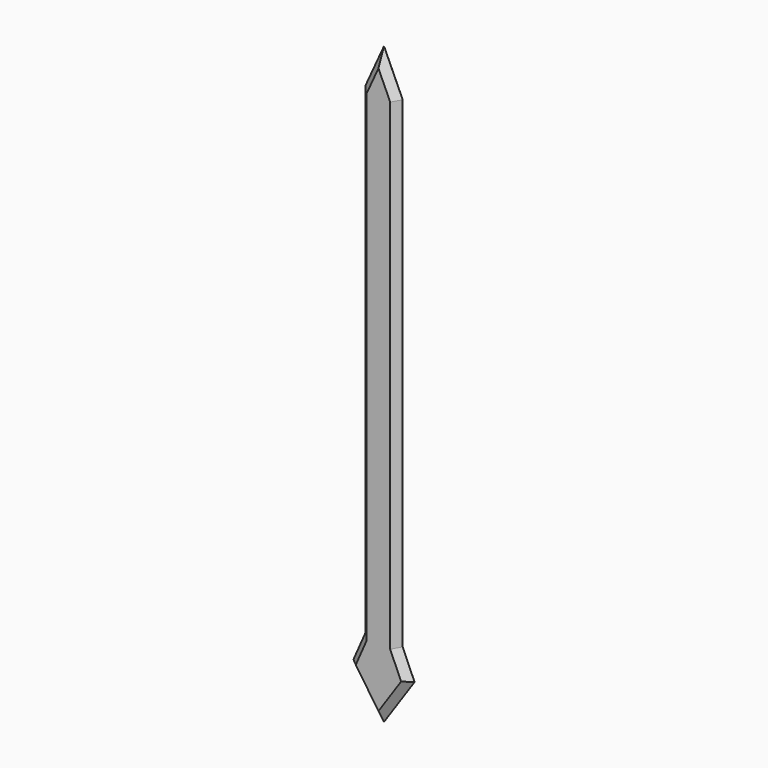
from build123d import *

# Parameters (mm, degrees)
F1_DEPTH = 6.35
F2_DEPTH = 6.35
F3_SIZE2 = 6.34999
F3_SIZE  = 6.34999


# Not quite as in the source:
# - a fillet or chamfer is up to 0.001 mm smaller than in the source, because OpenCascade refuses the exact size


with BuildPart() as f1:
    # F0 (on Front) → F1 (new body)
    with BuildSketch(Plane.XZ):
        Polygon((-17.139416188, 28.1973872334), (-27.9807504267, 3.4191238228), (0, -37.7674587071), (27.964355424, 3.4191238228), (17.08493568, 28.1973872334), (17.08493568, 469.1244959831), (0, 506.7884922028), (-17.139416188, 469.1244959831), align=None)
    extrude(amount=F1_DEPTH)

    # F2 (add): a face of the model
    f2_faces = [f1.faces().sort_by_distance(p)[0] for p in [
        (-0.0248835797, 0, 225.9211420486),
    ]]
    extrude(f2_faces, amount=F2_DEPTH)

    # F3 (size 6.35 and 6.35 in the source; OpenCascade refuses exactly that, so slightly less here)
    f3_edges = [f1.edges().sort_by_distance(p)[0] for p in [
        (-22.560083, -6.35, 15.808256),
        (-13.990375, -6.35, -17.174167),
        (13.982178, -6.35, -17.174167),
        (22.524646, -6.35, 15.808256),
        (17.084936, -6.35, 248.660942),
        (8.542468, -6.35, 487.956494),
        (-8.569708, -6.35, 487.956494),
        (-17.139416, -6.35, 248.660942),
        (-22.560083, 6.35, 15.808256),
        (-13.990375, 6.35, -17.174167),
        (13.982178, 6.35, -17.174167),
        (22.524646, 6.35, 15.808256),
        (17.084936, 6.35, 248.660942),
        (8.542468, 6.35, 487.956494),
        (-8.569708, 6.35, 487.956494),
        (-17.139416, 6.35, 248.660942),
    ]]
    chamfer(f3_edges, length=F3_SIZE, length2=F3_SIZE2)


solid = f1.part
